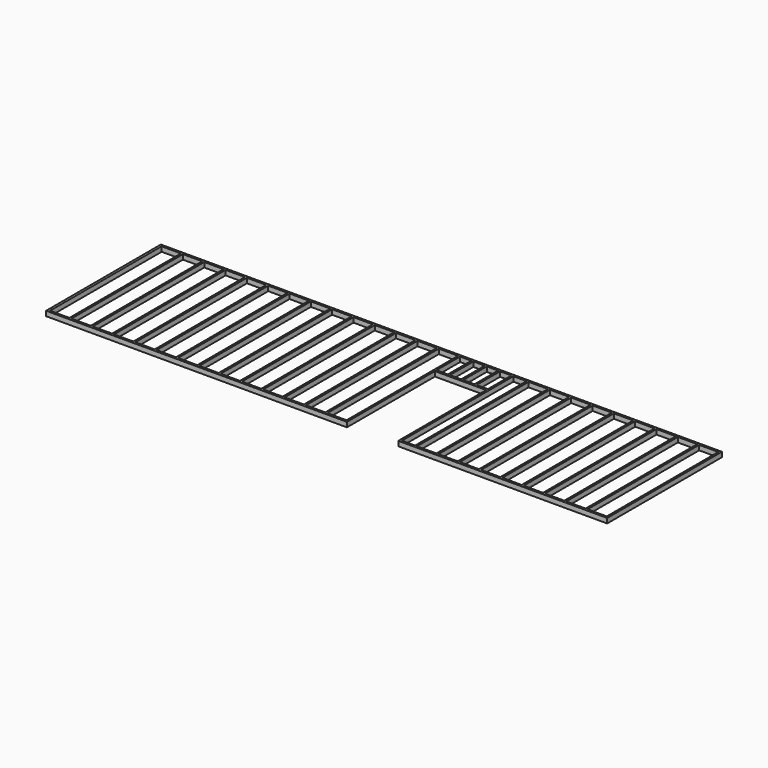
from build123d import *

# Parameters (mm, degrees)
F0_W     = 38.1
F0_H     = 2657.5512
F0_H_2   = 562.0512
F0_W_2   = 38.4048
F1_DEPTH = 92.075


# Not quite as in the source:
# - a feature names something its author has since deleted; it is built from what else it names


with BuildPart() as f1:
    # F0 (on Top) → F1 (new body)
    with BuildSketch(Plane.XY):
        Polygon((1365.1484, -1366.8756), (5346.6492, -1366.8756), (5346.6492, 1366.8756), (-5346.6492, 1366.8756), (-5346.6492, -1366.8756), (387.2484, -1366.8756), (387.2484, -1328.7756), (349.1484, -1328.7756), (-19.05, -1328.7756), (-57.15, -1328.7756), (-425.3484, -1328.7756), (-463.4484, -1328.7756), (-831.6468, -1328.7756), (-869.7468, -1328.7756), (-1237.9452, -1328.7756), (-1276.0452, -1328.7756), (-1644.2436, -1328.7756), (-1682.3436, -1328.7756), (-2050.542, -1328.7756), (-2088.642, -1328.7756), (-2456.8404, -1328.7756), (-2494.9404, -1328.7756), (-2863.1388, -1328.7756), (-2901.2388, -1328.7756), (-3269.4372, -1328.7756), (-3307.5372, -1328.7756), (-3675.7356, -1328.7756), (-3713.8356, -1328.7756), (-4082.034, -1328.7756), (-4120.134, -1328.7756), (-4488.3324, -1328.7756), (-4526.4324, -1328.7756), (-4894.6308, -1328.7756), (-4932.7308, -1328.7756), (-5300.9292, -1328.7756), (-5300.9292, 1328.7756), (-4932.7308, 1328.7756), (-4894.6308, 1328.7756), (-4526.4324, 1328.7756), (-4488.3324, 1328.7756), (-4120.134, 1328.7756), (-4082.034, 1328.7756), (-3713.8356, 1328.7756), (-3675.7356, 1328.7756), (-3307.5372, 1328.7756), (-3269.4372, 1328.7756), (-2901.2388, 1328.7756), (-2863.1388, 1328.7756), (-2494.9404, 1328.7756), (-2456.8404, 1328.7756), (-2088.642, 1328.7756), (-2050.542, 1328.7756), (-1682.3436, 1328.7756), (-1644.2436, 1328.7756), (-1276.0452, 1328.7756), (-1237.9452, 1328.7756), (-869.7468, 1328.7756), (-831.6468, 1328.7756), (-463.4484, 1328.7756), (-425.3484, 1328.7756), (-57.15, 1328.7756), (-19.05, 1328.7756), (349.1484, 1328.7756), (387.2484, 1328.7756), (603.0976, 1328.7756), (641.1976, 1328.7756), (856.996, 1328.7756), (895.4008, 1328.7756), (1111.1992, 1328.7756), (1149.2992, 1328.7756), (1365.1484, 1328.7756), (1403.2484, 1328.7756), (1654.911601016, 1328.7756), (1693.011601016, 1328.7756), (2061.210001016, 1328.7756), (2099.310001016, 1328.7756), (2467.508401016, 1328.7756), (2505.608401016, 1328.7756), (2873.806801016, 1328.7756), (2911.906801016, 1328.7756), (3280.105201016, 1328.7756), (3318.205201016, 1328.7756), (3686.403601016, 1328.7756), (3724.503601016, 1328.7756), (4092.702001016, 1328.7756), (4130.802001016, 1328.7756), (4499.000401016, 1328.7756), (4537.100401016, 1328.7756), (4905.298801016, 1328.7756), (4943.398801016, 1328.7756), (5308.5492, 1328.7756), (5308.5492, -1328.7756), (4943.398801016, -1328.7756), (4905.298801016, -1328.7756), (4537.100401016, -1328.7756), (4499.000401016, -1328.7756), (4130.802001016, -1328.7756), (4092.702001016, -1328.7756), (3724.503601016, -1328.7756), (3686.403601016, -1328.7756), (3318.205201016, -1328.7756), (3280.105201016, -1328.7756), (2911.906801016, -1328.7756), (2873.806801016, -1328.7756), (2505.608401016, -1328.7756), (2467.508401016, -1328.7756), (2099.310001016, -1328.7756), (2061.210001016, -1328.7756), (1693.011601016, -1328.7756), (1654.911601016, -1328.7756), (1403.2484, -1328.7756), (1365.1484, -1328.7756), align=None)
        with Locations((-4913.6808, 0)):
            Rectangle(F0_W, F0_H)
        with Locations((-4507.3824, 0)):
            Rectangle(F0_W, F0_H)
        with Locations((-4101.084, 0)):
            Rectangle(F0_W, F0_H)
        with Locations((-3694.7856, 0)):
            Rectangle(F0_W, F0_H)
        with Locations((-3288.4872, 0)):
            Rectangle(F0_W, F0_H)
        with Locations((-2882.1888, 0)):
            Rectangle(F0_W, F0_H)
        with Locations((-2475.8904, 0)):
            Rectangle(F0_W, F0_H)
        with Locations((-2069.592, 0)):
            Rectangle(F0_W, F0_H)
        with Locations((-1663.2936, 0)):
            Rectangle(F0_W, F0_H)
        with Locations((-1256.9952, 0)):
            Rectangle(F0_W, F0_H)
        with Locations((-850.6968, 0)):
            Rectangle(F0_W, F0_H)
        with Locations((-444.3984, 0)):
            Rectangle(F0_W, F0_H)
        Polygon((349.1484, -1328.7756), (387.2484, -1328.7756), (387.2484, 728.6244), (387.2484, 766.7244), (387.2484, 1328.7756), (349.1484, 1328.7756), align=None)
        Polygon((387.2484, 728.6244), (1365.1484, 728.6244), (1365.1484, 766.7244), (1149.2992, 766.7244), (1111.1992, 766.7244), (895.4008, 766.7244), (856.996, 766.7244), (641.1976, 766.7244), (603.0976, 766.7244), (387.2484, 766.7244), align=None)
        with Locations((622.1476, 1047.75)):
            Rectangle(F0_W, F0_H_2)
        with Locations((876.1984, 1047.75)):
            Rectangle(F0_W_2, F0_H_2)
        with Locations((1130.2492, 1047.75)):
            Rectangle(F0_W, F0_H_2)
        Polygon((1365.1484, 728.6244), (1365.1484, -1328.7756), (1403.2484, -1328.7756), (1403.2484, 1328.7756), (1365.1484, 1328.7756), (1365.1484, 766.7244), align=None)
        with Locations((1673.961601016, 0)):
            Rectangle(F0_W, F0_H)
        with Locations((2080.260001016, 0)):
            Rectangle(F0_W, F0_H)
        with Locations((2486.558401016, 0)):
            Rectangle(F0_W, F0_H)
        with Locations((2892.856801016, 0)):
            Rectangle(F0_W, F0_H)
        with Locations((3299.155201016, 0)):
            Rectangle(F0_W, F0_H)
        with Locations((3705.453601016, 0)):
            Rectangle(F0_W, F0_H)
        with Locations((4111.752001016, 0)):
            Rectangle(F0_W, F0_H)
        with Locations((4518.050401016, 0)):
            Rectangle(F0_W, F0_H)
        with Locations((4924.348801016, 0)):
            Rectangle(F0_W, F0_H)
        with Locations((-38.1, 0)):
            Rectangle(F0_W, F0_H)
    extrude(amount=F1_DEPTH)


solid = f1.part
